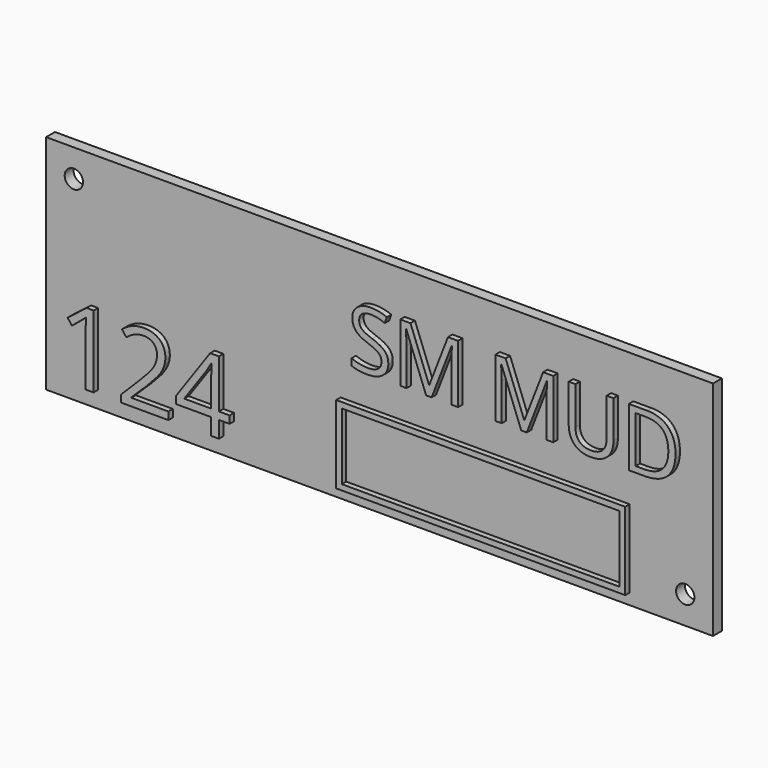
from build123d import *

# Parameters (mm, degrees)
F0_W         = 120
F0_H         = 40
F1_DEPTH     = 2
F3_D         = 3.3
F4_TEXT_SIZE = 14.7233618343
F5_DEPTH     = 1
F6_TEXT_SIZE = 18.1818181818
F7_DEPTH     = 1
F8_W         = 52
F8_H         = 14
F8_W_2       = 49.99999962
F8_H_2       = 11.99999962
F9_DEPTH     = 1


# Not quite as in the source:
# - Text() gives the source's letters only with a copy of the font that has no kerning and outlines rounded to 1/6400 em; it was checked with that copy


with BuildPart() as f1:
    # F0 (on Front) → F1 (new body)
    with BuildSketch(Plane.XZ):
        Rectangle(F0_W, F0_H)
    extrude(amount=F1_DEPTH)

    # F3 (through all)
    with Locations(Plane.XZ.offset(2)):
        with Locations((-55, 15), (55, -15)):
            Hole(F3_D / 2)

    # F4 (on face) → F5 (join)
    with BuildSketch(Plane.XZ.offset(2)):
        with Locations((-5, 2)):
            Text('SM MUD', F4_TEXT_SIZE, font='Open Sans', text_align=(TextAlign.LEFT, TextAlign.BOTTOM))
    extrude(amount=F5_DEPTH)

    # F6 (on face) → F7 (join)
    with BuildSketch(Plane.XZ.offset(2)):
        with Locations((-57, -17)):
            Text('124', F6_TEXT_SIZE, font='Open Sans', text_align=(TextAlign.LEFT, TextAlign.BOTTOM))
    extrude(amount=F7_DEPTH)

    # F8 (on face) → F9 (join)
    with BuildSketch(Plane.XZ.offset(2)):
        with Locations((19, -11)):
            Rectangle(F8_W, F8_H)
        with Locations((19, -11)):
            Rectangle(F8_W_2, F8_H_2, mode=Mode.SUBTRACT)
    extrude(amount=F9_DEPTH)


solid = f1.part
